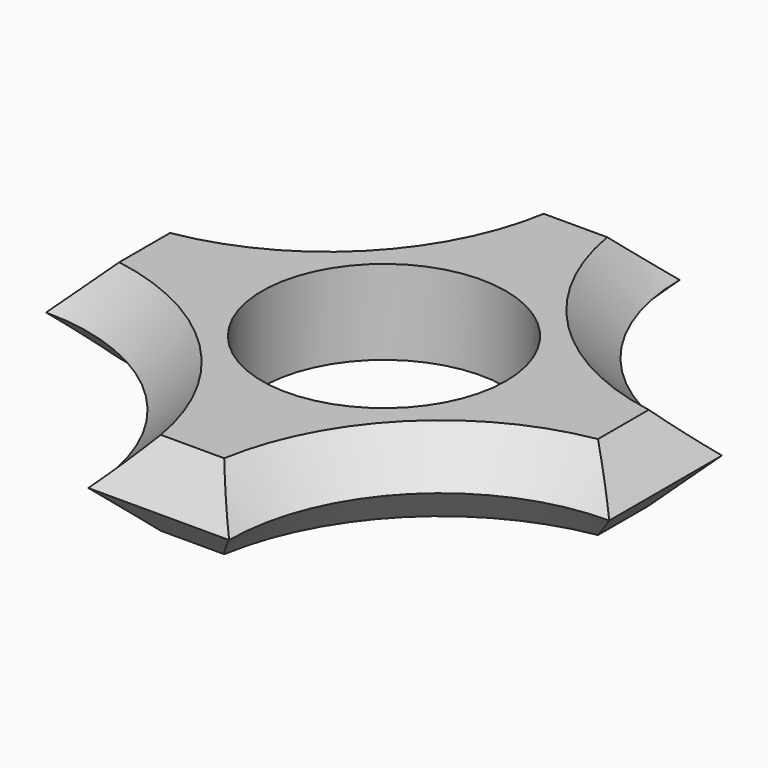
from build123d import *

# Parameters (mm, degrees)
F0_R     = 11
F1_DEPTH = 7.62
F2_SIZE  = 3.80999


# Not quite as in the source:
# - a fillet or chamfer is up to 0.001 mm smaller than in the source, because OpenCascade refuses the exact size


with BuildPart() as f1:
    # F0 (on Top) → F1 (new body)
    with BuildSketch(Plane.XY):
        with BuildLine():
            Line((6.35, 25.4), (-6.35, 25.4))
            ThreePointArc((-6.35, 25.4), (-11.9296158184, 11.9296158184), (-25.4, 6.35))
            Line((-25.4, 6.35), (-25.4, -6.35))
            ThreePointArc((-25.4, -6.35), (-11.9296158184, -11.9296158184), (-6.35, -25.4))
            Line((-6.35, -25.4), (6.35, -25.4))
            ThreePointArc((6.35, -25.4), (11.9296158184, -11.9296158184), (25.4, -6.35))
            Line((25.4, -6.35), (25.4, 6.35))
            ThreePointArc((25.4, 6.35), (11.9296158184, 11.9296158184), (6.35, 25.4))
        make_face()
        Circle(F0_R, mode=Mode.SUBTRACT)
    extrude(amount=F1_DEPTH)

    # F2 (size 3.81 in the source; OpenCascade refuses exactly that, so slightly less here)
    f2_edges = [f1.edges().sort_by_distance(p)[0] for p in [
        (11.929616, 11.929616, 7.62),
        (-11.929616, 11.929616, 7.62),
        (0, 25.4, 7.62),
        (25.4, 0, 7.62),
        (11.929616, -11.929616, 7.62),
        (0, -25.4, 7.62),
        (-11.929616, -11.929616, 7.62),
        (-25.4, 0, 7.62),
        (-11.929616, 11.929616, 0),
        (0, 25.4, 0),
        (11.929616, 11.929616, 0),
        (11.929616, -11.929616, 0),
        (25.4, 0, 0),
        (-11.929616, -11.929616, 0),
        (0, -25.4, 0),
        (-25.4, 0, 0),
    ]]
    chamfer(f2_edges, length=F2_SIZE)


solid = f1.part
